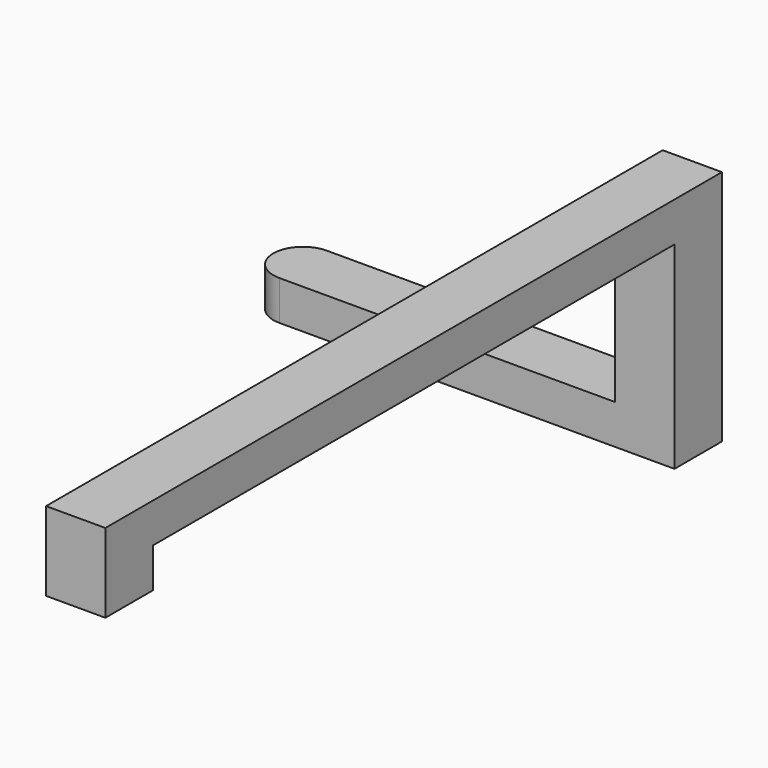
from build123d import *

# Parameters (mm, degrees)
F0_W     = 19.0500000055
F0_H     = 19.05
F1_DEPTH = 12.7
F2_DEPTH = 76.2
F3_W     = 19.05
F3_H     = 209.55
F4_DEPTH = 12.7
F3_H_2   = 19.05
F5_DEPTH = 25.4


# Not quite as in the source:
# - a feature names something its author has since deleted; it is built from what else it names


with BuildPart() as f1:
    # F0 (on Top) → F1 (new body)
    with BuildSketch(Plane.XY):
        with BuildLine():
            Line((46.7271760769, 7.14375), (-61.2228239231, 7.14375))
            ThreePointArc((-61.2228239231, 7.14375), (-70.7478239286, -2.3812499973), (-61.2228239286, -11.90625))
            Line((-61.2228239286, -11.90625), (46.7271760714, -11.90625))
            Line((46.7271760714, -11.90625), (46.7271760769, 7.14375))
        make_face()
        with Locations((56.2521760742, -2.38125)):
            Rectangle(F0_W, F0_H)
    extrude(amount=F1_DEPTH)

    # F0 (on Top) → F2 (join)
    with BuildSketch(Plane.XY):
        with Locations((56.2521760742, -2.38125)):
            Rectangle(F0_W, F0_H)
    extrude(amount=F2_DEPTH)

    # F3 (on face) → F4 (join)
    with BuildSketch(Plane.XY.offset(76.2)):
        with Locations((56.2521760742, -116.68125)):
            Rectangle(F3_W, F3_H)
    extrude(amount=-F4_DEPTH)

    # F3 (on face) → F5 (join)
    with BuildSketch(Plane.XY.offset(76.2)):
        with Locations((56.2521760742, -230.98125)):
            Rectangle(F3_W, F3_H_2)
    extrude(amount=-F5_DEPTH)


with BuildPart() as f6_1:
    # F6: copy of F1
    add(f1.part)


solid = f1.part
